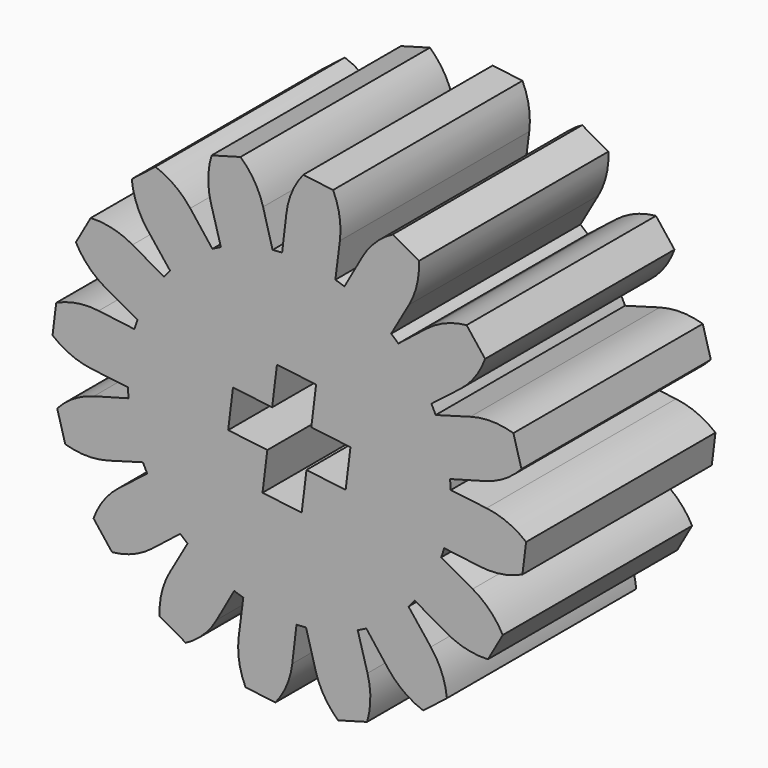
from build123d import *

# Parameters (mm, degrees)
F2_R            = 5.46
F3_DEPTH        = 8
F4_DEPTH        = 8
F4_COPIES_COUNT = 16
F6_DEPTH        = 25.4


# Not quite as in the source:
# - a pattern or mirror of a feature is missing from the dataset's text; its kind, count and spacing are read off the source's solid


with BuildPart() as f3:
    # F2 (on Front) → F3 (new body)
    with BuildSketch(Plane.XZ):
        Circle(F2_R)
    extrude(amount=F3_DEPTH)

    # F0 (on Front) → F4 (join, through all)
    with BuildSketch(Plane.XZ):
        with BuildLine():
            Line((1.4791617247, 7.8784603808), (0.4707348346, 8.0022796337))
            ThreePointArc((0.4707348346, 8.0022796337), (0.0898874426, 7.3746171039), (-0.099337312, 6.6652519091))
            Line((-0.099337312, 6.6652519091), (-0.2432709729, 5.4545778236))
            ThreePointArc((-0.2432709729, 5.4545778236), (0.6654030831, 5.4193024216), (1.5556197703, 5.2337030036))
            Line((1.5556197703, 5.2337030036), (1.7088476245, 6.4432359154))
            ThreePointArc((1.7088476245, 6.4432359154), (1.6968529376, 7.1773074522), (1.4791617247, 7.8784603808))
        make_face()
    f4 = extrude(amount=F4_DEPTH)

    # F4_copies: F4 ×16 about axis
    f4_copies_axis = Axis((0, 0, 0), (0, 1, 0))
    for i in range(1, F4_COPIES_COUNT):
        add(f4.rotate(f4_copies_axis, i * 360 / F4_COPIES_COUNT))

    # F5 (on Front) → F6 (cut)
    with BuildSketch(Plane.XZ):
        Polygon((0.7429432851, 0.5804516897), (0.9054348805, 1.9038466644), (0.2437373931, 1.9850924621), (-0.4179600943, 2.0663382598), (-0.5804516897, 0.7429432851), (-1.9038466644, 0.9054348805), (-1.9850924621, 0.2437373931), (-2.0663382598, -0.4179600943), (-0.7429432851, -0.5804516897), (-0.9054348805, -1.9038466644), (-0.2437373931, -1.9850924621), (0.4179600943, -2.0663382598), (0.5804516897, -0.7429432851), (1.9038466644, -0.9054348805), (1.9850924621, -0.2437373931), (2.0663382598, 0.4179600943), align=None)
    extrude(amount=F6_DEPTH, mode=Mode.SUBTRACT)


solid = f3.part
